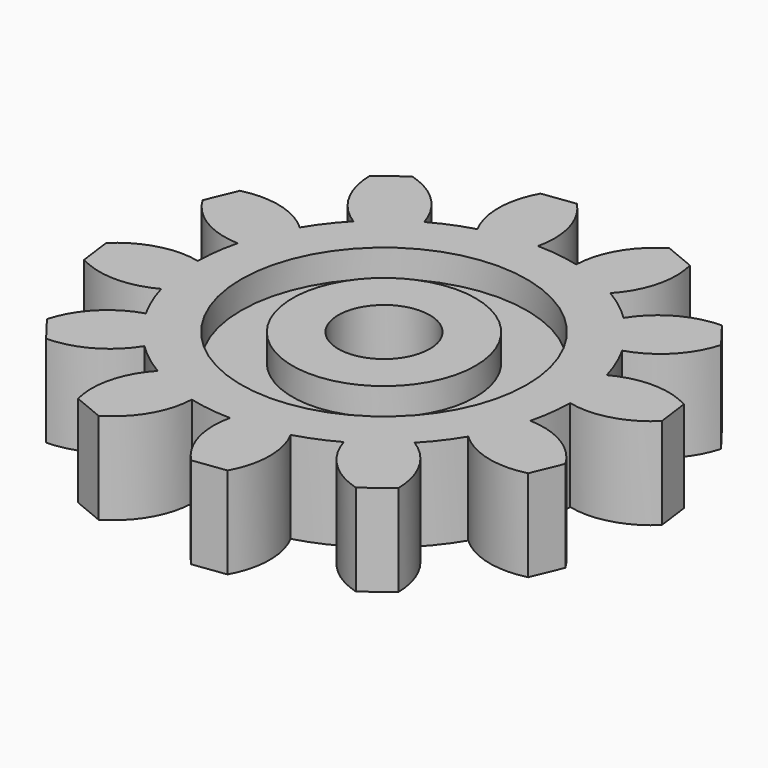
from build123d import *

# Parameters (mm, degrees)
F2_R     = 2.5
F4_DEPTH = 5
F5_COUNT = 12
F5_ANGLE = 330
F6_R     = 7.8035714286
F6_R_2   = 5
F7_DEPTH = 1.5
F8_START = 3.5
F8_DEPTH = 1.5


# Not quite as in the source:
# - a feature names something its author has since deleted; it is built from what else it names


with BuildPart() as f4:
    # F2 (on Top) → F4 (new body)
    with BuildSketch(Plane.XY):
        with BuildLine():
            ThreePointArc((-2.828404167, 9.9077602944), (-1.3448859448, 10.2154229467), (0.1677115736, 10.3022064147))
            ThreePointArc((0.1677115736, 10.3022064147), (0.1151870939, 12.4936954813), (-0.981879075, 14.3915439923))
            Line((-0.981879075, 14.3915439923), (-2.7763833168, 14.1552930269))
            ThreePointArc((-2.7763833168, 14.1552930269), (-3.3448685232, 12.0381705175), (-2.828404167, 9.9077602944))
        make_face()
        with BuildLine():
            ThreePointArc((-2.828404167, 9.9077602944), (-6.2056796493, -8.2251519301), (10.3035714286, 0))
            ThreePointArc((10.3035714286, 0), (7.3447808804, 7.2261869615), (0.1677115736, 10.3022064147))
            ThreePointArc((0.1677115736, 10.3022064147), (-1.3448859448, 10.2154229467), (-2.828404167, 9.9077602944))
        make_face()
        Circle(F2_R, mode=Mode.SUBTRACT)
    extrude(amount=F4_DEPTH)

    # F5: F4 ×12 about axis
    f5_axis = Axis((0, 0, 30.7848658413), (0, 0, 1))


with BuildPart() as f4_1:
    add(f4.part)
    for i in range(1, F5_COUNT):
        add(f4.part.rotate(f5_axis, i * F5_ANGLE / (F5_COUNT - 1)))

    # F6 (on Top) → F7 (cut)
    with BuildSketch(Plane.XY):
        Circle(F6_R)
        Circle(F6_R_2, mode=Mode.SUBTRACT)
    extrude(amount=F7_DEPTH, mode=Mode.SUBTRACT)

    # F6 (on Top) → F8 (cut)
    with BuildSketch(Plane.XY.offset(F8_START)):
        Circle(F6_R)
        Circle(F6_R_2, mode=Mode.SUBTRACT)
    extrude(amount=F8_DEPTH, mode=Mode.SUBTRACT)


solid = f4_1.part
